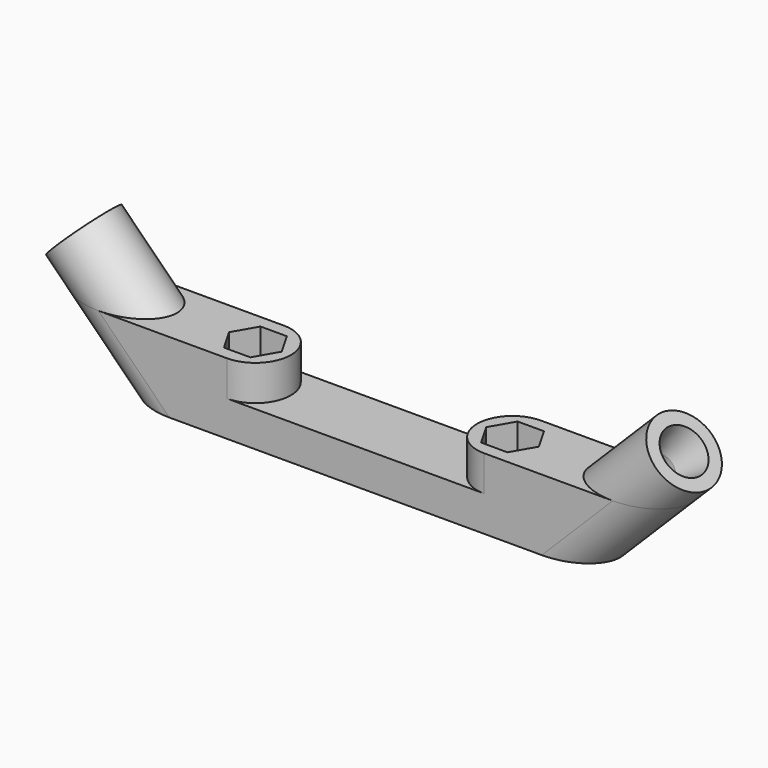
from build123d import *

# Parameters (mm, degrees)
F1_DEPTH  = 4
F2_R      = 3.99999
F4_DEPTH  = 8
F6_DEPTH  = 4
F9_R      = 4
F10_DEPTH = 6.851053331
F12_SIZE2 = 1
F12_SIZE  = 3.7320508076


# Not quite as in the source:
# - a fillet or chamfer is up to 0.001 mm smaller than in the source, because OpenCascade refuses the exact size


with BuildPart() as f1:
    # F0 (on Front) → F1 (new body, symmetric)
    with BuildSketch(Plane.XZ):
        Polygon((-26.6568542495, 0), (0, 0), (0, 8), (-34.6568542495, 8), align=None)
    extrude(amount=F1_DEPTH, both=True)

    # F2 (radius 4 in the source; OpenCascade refuses exactly that, so slightly less here)
    f2_edges = [f1.edges().sort_by_distance(p)[0] for p in [
        (-30.656854, 4, 4),
        (-30.656854, -4, 4),
    ]]
    fillet(f2_edges, radius=F2_R)

    # F3 (on face) → F4 (cut, through all)
    with BuildSketch(Plane.XY.offset(8)):
        Polygon((-11.5266461137, 0), (-13.0133230568, 2.575), (-15.9866769432, 2.575), (-17.4733538863, 0), (-15.9866769432, -2.575), (-13.0133230568, -2.575), align=None)
    extrude(amount=-F4_DEPTH, mode=Mode.SUBTRACT)

    # F5 (on face) → F6 (cut)
    with BuildSketch(Plane.XY.offset(8)):
        with BuildLine():
            ThreePointArc((-14.5, 4), (-10.5, 0), (-14.5, -4))
            Line((-14.5, -4), (0, -4))
            Line((0, -4), (0, 4))
            Line((0, 4), (-14.5, 4))
        make_face()
    extrude(amount=-F6_DEPTH, mode=Mode.SUBTRACT)

    # F9 (on line) → F10 (join, symmetric)
    with BuildSketch(Plane(origin=(-18.5, 0, 18.5), x_dir=(0, 1, 0), z_dir=(0.7071067812, 0, -0.7071067812))):
        with Locations((0, -14.8492424049)):
            Circle(F9_R)
    extrude(amount=F10_DEPTH, both=True)

    # F7 (on Front) → F11 (revolve, cut)
    with BuildSketch(Plane.XZ):
        Polygon((-11.4302859145, -11.8147781158), (-10.3077538993, -10.6922461007), (-44.6173825807, 23.6173825807), (-45.7399145958, 22.4948505656), align=None)
    revolve(axis=Axis((-27.46256824, 0, 6.46256824), (-0.7071067812, 0, 0.7071067812)), mode=Mode.SUBTRACT)

    # F12
    f12_edges = [f1.edges().sort_by_distance(p)[0] for p in [
        (-32.721894, 0, 13.966958),
    ]]
    f12_side = f1.faces().sort_by_distance((-25.685621, 0, 6.930685))[0]
    chamfer(f12_edges, length=F12_SIZE, length2=F12_SIZE2, reference=f12_side)

    # F13: F1 across face


with BuildPart() as f1_1:
    add(f1.part)
    add(f1.part.mirror(Plane(origin=(0, 0, 2), x_dir=(0, 1, 0), z_dir=(1, 0, 0))))


solid = f1_1.part
